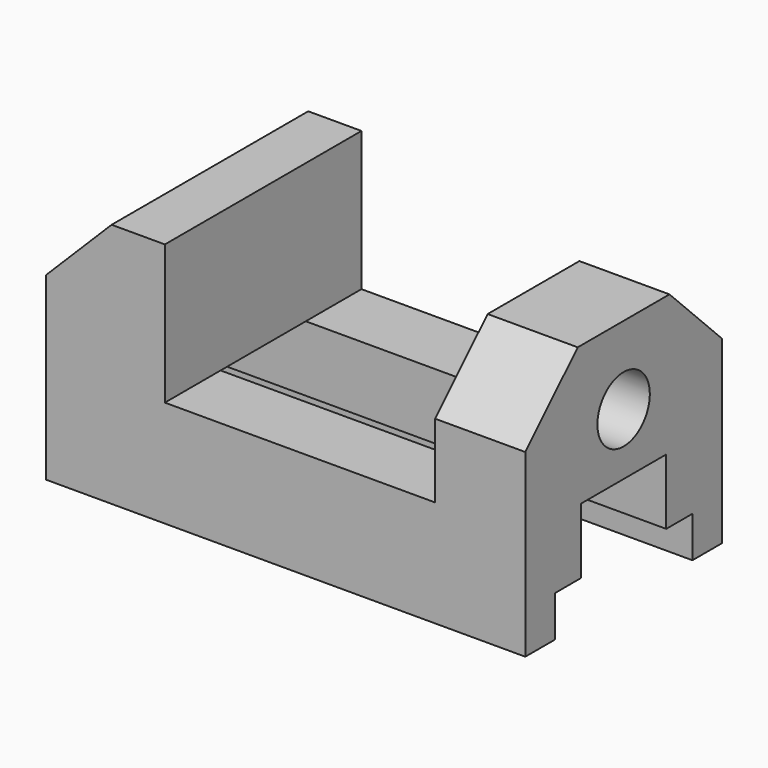
from build123d import *

# Parameters (mm, degrees)
F0_W      = 117
F0_H      = 60
F1_DEPTH  = 60
F2_W      = 66
F2_H      = 34
F3_DEPTH  = 60
F5_DEPTH  = 60
F7_DEPTH  = 22
F10_DEPTH = 117.001
F11_R     = 8
F12_DEPTH = 22


# Not quite as in the source:
# - a pattern or mirror of a feature is missing from the dataset's text; its kind, count and spacing are read off the source's solid


with BuildPart() as f1:
    # F0 (on Front) → F1 (new body)
    with BuildSketch(Plane.XZ):
        Rectangle(F0_W, F0_H)
    extrude(amount=F1_DEPTH)

    # F2 (on face) → F3 (cut, through all)
    with BuildSketch(Plane.XZ.offset(60)):
        with Locations((3.5, 13)):
            Rectangle(F2_W, F2_H)
    extrude(amount=-F3_DEPTH, mode=Mode.SUBTRACT)

    # F4 (on face) → F5 (cut, through all)
    with BuildSketch(Plane.XZ.offset(60)):
        Polygon((-58.5, 30), (-58.5, 14), (-42.5, 30), align=None)
    extrude(amount=-F5_DEPTH, mode=Mode.SUBTRACT)

    # F6 (on face) → F7 (cut, through all)
    with BuildSketch(Plane.YZ.offset(58.5)):
        Polygon((-60, 30), (-60, 14), (-44, 30), align=None)
    f7 = extrude(amount=-F7_DEPTH, mode=Mode.SUBTRACT)

    # F7_copies: F7 across plane
    add(f7.mirror(Plane.ZX.offset(-30)), mode=Mode.SUBTRACT)

    # F9 (on face) → F10 (cut, through all)
    with BuildSketch(Plane.YZ.offset(58.5)):
        Polygon((-51, -20), (-51, -30), (-9, -30), (-9, -20), (-17, -20), (-17, -4), (-43, -4), (-43, -20), align=None)
    extrude(amount=-F10_DEPTH, mode=Mode.SUBTRACT)

    # F11 (on face) → F12 (cut, through all)
    with BuildSketch(Plane.YZ.offset(58.5)):
        with Locations((-30, 11)):
            Circle(F11_R)
    extrude(amount=-F12_DEPTH, mode=Mode.SUBTRACT)


solid = f1.part
